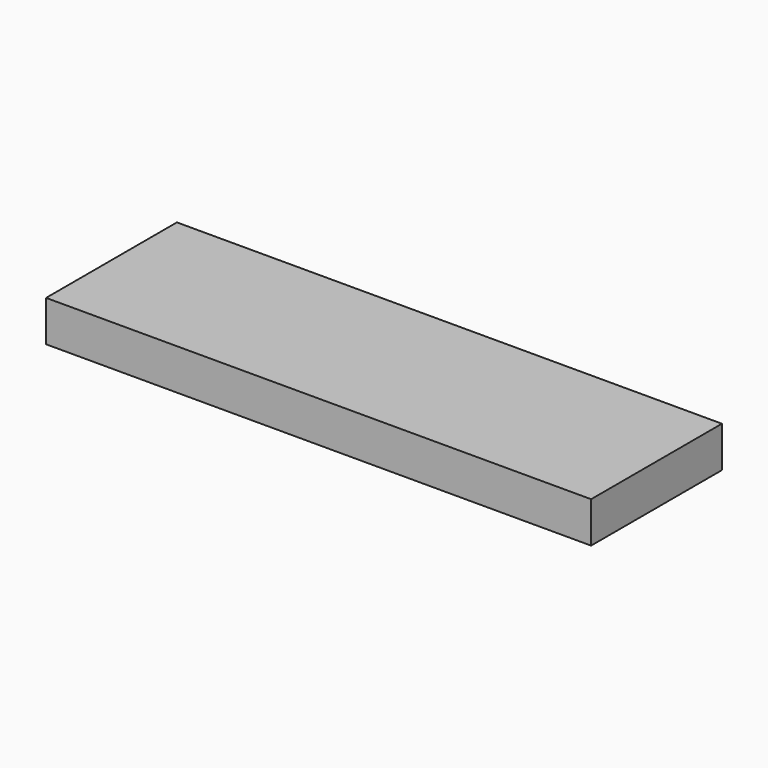
from build123d import *

# Parameters (mm, degrees)
F0_W     = 508
F0_H     = 152.4
F1_DEPTH = 38.1


# Not quite as in the source:
# - a feature of the source that left no trace in its solid (it failed there, or was rolled back) is left out


with BuildPart() as f1:
    # F0 (on Top) → F1 (new body)
    with BuildSketch(Plane.XY):
        Rectangle(F0_W, F0_H)
    extrude(amount=F1_DEPTH)


solid = f1.part
